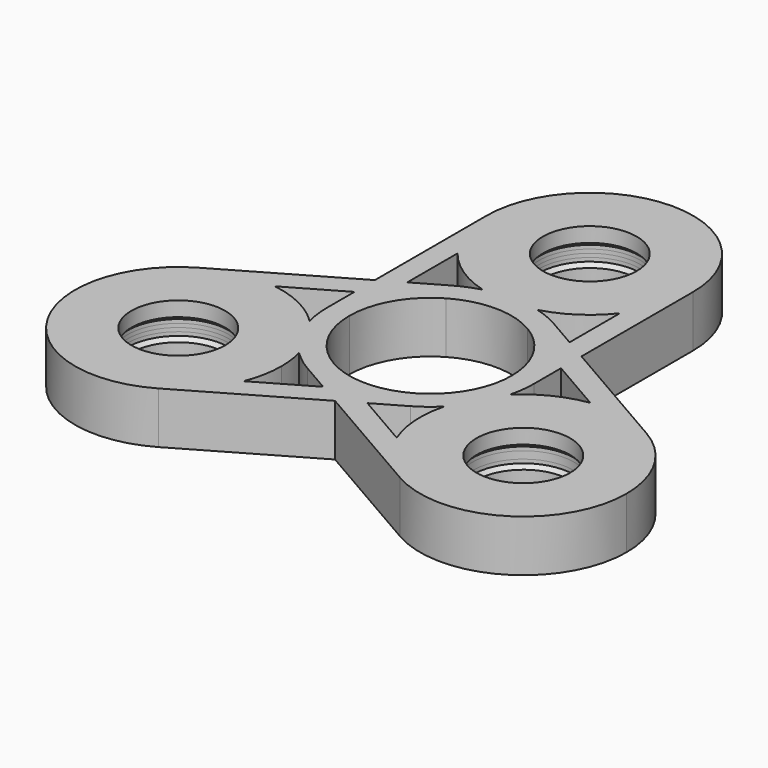
from build123d import *

# Parameters (mm, degrees)
F0_R         = 6.85
F0_R_2       = 6.35
F1_DEPTH     = 3.5
F2_DEPTH     = 0.5
F3_S5_R      = 6.85
F3_T6_DEPTH  = 12
F3_S11_R     = 6.85
F3_T12_DEPTH = 12
F3_S17_R     = 6.85
F3_T18_DEPTH = 12
F3_S23_R     = 6.85
F3_T24_DEPTH = 12
F3_S29_R     = 6.85
F3_T30_DEPTH = 12
F3_S35_R     = 6.85
F3_T36_DEPTH = 12


# Not quite as in the source:
# - a fillet or chamfer that OpenCascade refuses, or shapes differently, is made with other operations: its cross-section is extruded or revolved along the edge and cut away or added


with BuildPart() as f1:
    # F0 (on Top) → F1 (new body, symmetric)
    with BuildSketch(Plane.XY):
        with BuildLine():
            ThreePointArc((-11, 27), (0, 16), (11, 27))
            ThreePointArc((11, 27), (0, 38), (-11, 27))
        make_face()
        with Locations((0, 27)):
            Circle(F0_R, mode=Mode.SUBTRACT)
        with BuildLine():
            ThreePointArc((-28.882686, -3.973721), (-32.908965, -19), (-17.882686, -23.026279))
            ThreePointArc((-17.882686, -23.026279), (-13.856406, -19), (-12.382686, -13.5))
            ThreePointArc((-12.382686, -13.5), (-17.882686, -3.973721), (-28.882686, -3.973721))
        make_face()
        with Locations((-23.382686, -13.5)):
            Circle(F0_R, mode=Mode.SUBTRACT)
        with BuildLine():
            ThreePointArc((34.382686, -13.5), (32.908965, -8), (28.882686, -3.973721))
            ThreePointArc((28.882686, -3.973721), (13.856406, -8), (17.882686, -23.026279))
            ThreePointArc((17.882686, -23.026279), (28.882686, -23.026279), (34.382686, -13.5))
        make_face()
        with Locations((23.382686, -13.5)):
            Circle(F0_R, mode=Mode.SUBTRACT)
        with BuildLine():
            Line((11, 27), (11, 18.339746))
            ThreePointArc((11, 18.339746), (13.228757, 22.417424), (14, 27))
            ThreePointArc((14, 27), (0, 41), (-14, 27))
            ThreePointArc((-14, 27), (-13.228757, 22.417424), (-11, 18.339746))
            Line((-11, 18.339746), (-11, 27))
            ThreePointArc((-11, 27), (0, 38), (11, 27))
        make_face()
        with BuildLine():
            ThreePointArc((-16.382686, -25.624356), (-12.799681, -22.665151), (-10.382686, -18.696152))
            Line((-10.382686, -18.696152), (-17.882686, -23.026279))
            ThreePointArc((-17.882686, -23.026279), (-32.908965, -19), (-28.882686, -3.973721))
            Line((-28.882686, -3.973721), (-21.382686, 0.356406))
            ThreePointArc((-21.382686, 0.356406), (-26.028437, 0.247727), (-30.382686, -1.375644))
            ThreePointArc((-30.382686, -1.375644), (-35.507042, -20.5), (-16.382686, -25.624356))
        make_face()
        with BuildLine():
            ThreePointArc((30.382686, -1.375644), (26.028437, 0.247727), (21.382686, 0.356406))
            Line((21.382686, 0.356406), (28.882686, -3.973721))
            ThreePointArc((28.882686, -3.973721), (32.908965, -8), (34.382686, -13.5))
            ThreePointArc((34.382686, -13.5), (28.882686, -23.026279), (17.882686, -23.026279))
            Line((17.882686, -23.026279), (10.382686, -18.696152))
            ThreePointArc((10.382686, -18.696152), (12.799681, -22.665151), (16.382686, -25.624356))
            ThreePointArc((16.382686, -25.624356), (30.382686, -25.624356), (37.382686, -13.5))
            ThreePointArc((37.382686, -13.5), (35.507042, -6.5), (30.382686, -1.375644))
        make_face()
        with Locations((0, 27)):
            Circle(F0_R)
        with Locations((0, 27)):
            Circle(F0_R_2, mode=Mode.SUBTRACT)
        with Locations((-23.382686, -13.5)):
            Circle(F0_R)
        with Locations((-23.382686, -13.5)):
            Circle(F0_R_2, mode=Mode.SUBTRACT)
        with Locations((23.382686, -13.5)):
            Circle(F0_R)
        with Locations((23.382686, -13.5)):
            Circle(F0_R_2, mode=Mode.SUBTRACT)
        with BuildLine():
            ThreePointArc((-3.708099, 13.5), (0, 14), (3.708099, 13.5))
            ThreePointArc((3.708099, 13.5), (7.741953, 15.335431), (11, 18.339746))
            Line((11, 18.339746), (11, 27))
            ThreePointArc((11, 27), (0, 16), (-11, 27))
            Line((-11, 27), (-11, 18.339746))
            ThreePointArc((-11, 18.339746), (-7.741953, 15.335431), (-3.708099, 13.5))
        make_face()
        with BuildLine():
            ThreePointArc((-9.382686, -13.5), (-9.496803, -11.716113), (-9.837293, -9.961308))
            ThreePointArc((-9.837293, -9.961308), (-12.124356, -7), (-13.545393, -3.538692))
            ThreePointArc((-13.545393, -3.538692), (-17.151849, -0.962988), (-21.382686, 0.356406))
            Line((-21.382686, 0.356406), (-28.882686, -3.973721))
            ThreePointArc((-28.882686, -3.973721), (-17.882686, -3.973721), (-12.382686, -13.5))
            ThreePointArc((-12.382686, -13.5), (-13.856406, -19), (-17.882686, -23.026279))
            Line((-17.882686, -23.026279), (-10.382686, -18.696152))
            ThreePointArc((-10.382686, -18.696152), (-9.634959, -16.145751), (-9.382686, -13.5))
        make_face()
        with BuildLine():
            ThreePointArc((21.382686, 0.356406), (17.151849, -0.962988), (13.545393, -3.538692))
            ThreePointArc((13.545393, -3.538692), (12.124356, -7), (9.837293, -9.961308))
            ThreePointArc((9.837293, -9.961308), (9.409897, -14.372443), (10.382686, -18.696152))
            Line((10.382686, -18.696152), (17.882686, -23.026279))
            ThreePointArc((17.882686, -23.026279), (13.856406, -8), (28.882686, -3.973721))
            Line((28.882686, -3.973721), (21.382686, 0.356406))
        make_face()
        with BuildLine():
            ThreePointArc((-5.5, 9.526279), (0, 11), (5.5, 9.526279))
            Line((5.5, 9.526279), (11, 6.350853))
            Line((11, 6.350853), (11, 8.660254))
            ThreePointArc((11, 8.660254), (9.165151, 10.583005), (7, 12.124356))
            ThreePointArc((7, 12.124356), (5.39805, 12.917471), (3.708099, 13.5))
            ThreePointArc((3.708099, 13.5), (0, 13), (-3.708099, 13.5))
            ThreePointArc((-3.708099, 13.5), (-5.39805, 12.917471), (-7, 12.124356))
            ThreePointArc((-7, 12.124356), (-9.165151, 10.583005), (-11, 8.660254))
            Line((-11, 8.660254), (-11, 6.350853))
            Line((-11, 6.350853), (-5.5, 9.526279))
        make_face()
        with BuildLine():
            Line((11, 6.350853), (11, 0))
            ThreePointArc((11, 0), (9.526279, -5.5), (5.5, -9.526279))
            Line((5.5, -9.526279), (0, -12.701706))
            Line((0, -12.701706), (2, -13.856406))
            ThreePointArc((2, -13.856406), (4.582576, -13.228757), (7, -12.124356))
            ThreePointArc((7, -12.124356), (8.487833, -11.133584), (9.837293, -9.961308))
            ThreePointArc((9.837293, -9.961308), (11.25833, -6.5), (13.545393, -3.538692))
            ThreePointArc((13.545393, -3.538692), (13.885883, -1.783887), (14, 0))
            ThreePointArc((14, 0), (13.747727, 2.645751), (13, 5.196152))
            Line((13, 5.196152), (11, 6.350853))
        make_face()
        with BuildLine():
            Line((0, -12.701706), (-5.5, -9.526279))
            ThreePointArc((-5.5, -9.526279), (-9.526279, -5.5), (-11, 0))
            Line((-11, 0), (-11, 6.350853))
            Line((-11, 6.350853), (-13, 5.196152))
            ThreePointArc((-13, 5.196152), (-13.747727, 2.645751), (-14, 0))
            ThreePointArc((-14, 0), (-13.885883, -1.783887), (-13.545393, -3.538692))
            ThreePointArc((-13.545393, -3.538692), (-11.25833, -6.5), (-9.837293, -9.961308))
            ThreePointArc((-9.837293, -9.961308), (-8.487833, -11.133584), (-7, -12.124356))
            ThreePointArc((-7, -12.124356), (-4.582576, -13.228757), (-2, -13.856406))
            Line((-2, -13.856406), (0, -12.701706))
        make_face()
        with BuildLine():
            Line((-14, 8.082904), (-11, 9.814955))
            Line((-11, 9.814955), (-11, 18.339746))
            ThreePointArc((-11, 18.339746), (-13.228757, 22.417424), (-14, 27))
            Line((-14, 27), (-14, 8.082904))
        make_face()
        with BuildLine():
            Line((-21.382686, 0.356406), (-14, 4.618802))
            Line((-14, 4.618802), (-14, 8.082904))
            Line((-14, 8.082904), (-30.382686, -1.375644))
            ThreePointArc((-30.382686, -1.375644), (-26.028437, 0.247727), (-21.382686, 0.356406))
        make_face()
        with BuildLine():
            Line((0, -16.165808), (-3, -14.433757))
            Line((-3, -14.433757), (-10.382686, -18.696152))
            ThreePointArc((-10.382686, -18.696152), (-12.799681, -22.665151), (-16.382686, -25.624356))
            Line((-16.382686, -25.624356), (0, -16.165808))
        make_face()
        with BuildLine():
            Line((10.382686, -18.696152), (3, -14.433757))
            Line((3, -14.433757), (0, -16.165808))
            Line((0, -16.165808), (16.382686, -25.624356))
            ThreePointArc((16.382686, -25.624356), (12.799681, -22.665151), (10.382686, -18.696152))
        make_face()
        with BuildLine():
            Line((14, 8.082904), (14, 4.618802))
            Line((14, 4.618802), (21.382686, 0.356406))
            ThreePointArc((21.382686, 0.356406), (26.028437, 0.247727), (30.382686, -1.375644))
            Line((30.382686, -1.375644), (14, 8.082904))
        make_face()
        with BuildLine():
            Line((11, 18.339746), (11, 9.814955))
            Line((11, 9.814955), (14, 8.082904))
            Line((14, 8.082904), (14, 27))
            ThreePointArc((14, 27), (13.228757, 22.417424), (11, 18.339746))
        make_face()
        with BuildLine():
            Line((-14, 4.618802), (-13, 5.196152))
            ThreePointArc((-13, 5.196152), (-12.124356, 7), (-11, 8.660254))
            Line((-11, 8.660254), (-11, 9.814955))
            Line((-11, 9.814955), (-14, 8.082904))
            Line((-14, 8.082904), (-14, 4.618802))
        make_face()
        with BuildLine():
            Line((11, 9.814955), (11, 8.660254))
            ThreePointArc((11, 8.660254), (12.124356, 7), (13, 5.196152))
            Line((13, 5.196152), (14, 4.618802))
            Line((14, 4.618802), (14, 8.082904))
            Line((14, 8.082904), (11, 9.814955))
        make_face()
        with BuildLine():
            ThreePointArc((2, -13.856406), (0, -14), (-2, -13.856406))
            Line((-2, -13.856406), (-3, -14.433757))
            Line((-3, -14.433757), (0, -16.165808))
            Line((0, -16.165808), (3, -14.433757))
            Line((3, -14.433757), (2, -13.856406))
        make_face()
        with BuildLine():
            ThreePointArc((-11, 0), (-9.526279, 5.5), (-5.5, 9.526279))
            Line((-5.5, 9.526279), (-11, 6.350853))
            Line((-11, 6.350853), (-11, 0))
        make_face()
        with BuildLine():
            ThreePointArc((5.5, 9.526279), (9.526279, 5.5), (11, 0))
            Line((11, 0), (11, 6.350853))
            Line((11, 6.350853), (5.5, 9.526279))
        make_face()
        with BuildLine():
            Line((0, -12.701706), (5.5, -9.526279))
            ThreePointArc((5.5, -9.526279), (0, -11), (-5.5, -9.526279))
            Line((-5.5, -9.526279), (0, -12.701706))
        make_face()
        with BuildLine():
            ThreePointArc((-3.708099, 13.5), (0, 13), (3.708099, 13.5))
            ThreePointArc((3.708099, 13.5), (0, 14), (-3.708099, 13.5))
        make_face()
        with BuildLine():
            ThreePointArc((-13.545393, -3.538692), (-12.124356, -7), (-9.837293, -9.961308))
            ThreePointArc((-9.837293, -9.961308), (-11.25833, -6.5), (-13.545393, -3.538692))
        make_face()
        with BuildLine():
            ThreePointArc((9.837293, -9.961308), (12.124356, -7), (13.545393, -3.538692))
            ThreePointArc((13.545393, -3.538692), (11.25833, -6.5), (9.837293, -9.961308))
        make_face()
        with BuildLine():
            Line((-13, 5.196152), (-11, 6.350853))
            Line((-11, 6.350853), (-11, 8.660254))
            ThreePointArc((-11, 8.660254), (-12.124356, 7), (-13, 5.196152))
        make_face()
        with BuildLine():
            Line((11, 8.660254), (11, 6.350853))
            Line((11, 6.350853), (13, 5.196152))
            ThreePointArc((13, 5.196152), (12.124356, 7), (11, 8.660254))
        make_face()
        with BuildLine():
            Line((2, -13.856406), (0, -12.701706))
            Line((0, -12.701706), (-2, -13.856406))
            ThreePointArc((-2, -13.856406), (0, -14), (2, -13.856406))
        make_face()
        with BuildLine():
            Line((-11, 9.814955), (-11, 8.660254))
            ThreePointArc((-11, 8.660254), (-9.165151, 10.583005), (-7, 12.124356))
            Line((-7, 12.124356), (-11, 9.814955))
        make_face()
        with BuildLine():
            ThreePointArc((-14, 0), (-13.747727, 2.645751), (-13, 5.196152))
            Line((-13, 5.196152), (-14, 4.618802))
            Line((-14, 4.618802), (-14, 0))
        make_face()
        with BuildLine():
            ThreePointArc((7, 12.124356), (9.165151, 10.583005), (11, 8.660254))
            Line((11, 8.660254), (11, 9.814955))
            Line((11, 9.814955), (7, 12.124356))
        make_face()
        with BuildLine():
            ThreePointArc((7, -12.124356), (4.582576, -13.228757), (2, -13.856406))
            Line((2, -13.856406), (3, -14.433757))
            Line((3, -14.433757), (7, -12.124356))
        make_face()
        with BuildLine():
            Line((14, 4.618802), (13, 5.196152))
            ThreePointArc((13, 5.196152), (13.747727, 2.645751), (14, 0))
            Line((14, 0), (14, 4.618802))
        make_face()
        with BuildLine():
            Line((-3, -14.433757), (-2, -13.856406))
            ThreePointArc((-2, -13.856406), (-4.582576, -13.228757), (-7, -12.124356))
            Line((-7, -12.124356), (-3, -14.433757))
        make_face()
    extrude(amount=F1_DEPTH, both=True)

    # F0 (on Top) → F2 (cut, symmetric)
    with BuildSketch(Plane.XY):
        with Locations((0, 27)):
            Circle(F0_R)
        with Locations((0, 27)):
            Circle(F0_R_2, mode=Mode.SUBTRACT)
        with Locations((-23.382686, -13.5)):
            Circle(F0_R)
        with Locations((-23.382686, -13.5)):
            Circle(F0_R_2, mode=Mode.SUBTRACT)
        with Locations((23.382686, -13.5)):
            Circle(F0_R)
        with Locations((23.382686, -13.5)):
            Circle(F0_R_2, mode=Mode.SUBTRACT)
    extrude(amount=F2_DEPTH, both=True, mode=Mode.SUBTRACT)

    # F3: chamfer of 1 on 6 edges, made by hand


with BuildPart() as f3_tool2:
    # F3_s3 → F3_t4 (revolve)
    with BuildSketch(Plane.XZ.offset(-27)):
        Polygon((6.35, 1.5), (7.35, 0.5), (6.35, 0.5), align=None)
    revolve(axis=Axis((0, 27, 0.5), (0, 0, 1)))

    # F3_s5 → F3_t6 (intersect, symmetric)
    with BuildSketch(Plane.XY.offset(1)):
        with Locations((0, 27)):
            Circle(F3_S5_R)
    extrude(amount=F3_T6_DEPTH, both=True, mode=Mode.INTERSECT)


with BuildPart() as f1_1:
    add(f1.part)

    # F3_t1: cut F3_tool2
    add(f3_tool2.part, mode=Mode.SUBTRACT)


with BuildPart() as f3_tool8:
    # F3_s9 → F3_t10 (revolve)
    with BuildSketch(Plane.XZ.offset(-27)):
        Polygon((7.35, -0.5), (6.35, -1.5), (6.35, -0.5), align=None)
    revolve(axis=Axis((0, 27, -0.5), (0, 0, 1)))

    # F3_s11 → F3_t12 (intersect, symmetric)
    with BuildSketch(Plane.XY.offset(-1)):
        with Locations((0, 27)):
            Circle(F3_S11_R)
    extrude(amount=F3_T12_DEPTH, both=True, mode=Mode.INTERSECT)


with BuildPart() as f1_2:
    add(f1_1.part)

    # F3_t7: cut F3_tool8
    add(f3_tool8.part, mode=Mode.SUBTRACT)


with BuildPart() as f3_tool14:
    # F3_s15 → F3_t16 (revolve)
    with BuildSketch(Plane.XZ.offset(13.5)):
        Polygon((29.732686, 1.5), (30.732686, 0.5), (29.732686, 0.5), align=None)
    revolve(axis=Axis((23.382686, -13.5, 0.5), (0, 0, 1)))

    # F3_s17 → F3_t18 (intersect, symmetric)
    with BuildSketch(Plane.XY.offset(1)):
        with Locations((23.382686, -13.5)):
            Circle(F3_S17_R)
    extrude(amount=F3_T18_DEPTH, both=True, mode=Mode.INTERSECT)


with BuildPart() as f1_3:
    add(f1_2.part)

    # F3_t13: cut F3_tool14
    add(f3_tool14.part, mode=Mode.SUBTRACT)


with BuildPart() as f3_tool20:
    # F3_s21 → F3_t22 (revolve)
    with BuildSketch(Plane.XZ.offset(13.5)):
        Polygon((30.732686, -0.5), (29.732686, -1.5), (29.732686, -0.5), align=None)
    revolve(axis=Axis((23.382686, -13.5, -0.5), (0, 0, 1)))

    # F3_s23 → F3_t24 (intersect, symmetric)
    with BuildSketch(Plane.XY.offset(-1)):
        with Locations((23.382686, -13.5)):
            Circle(F3_S23_R)
    extrude(amount=F3_T24_DEPTH, both=True, mode=Mode.INTERSECT)


with BuildPart() as f1_4:
    add(f1_3.part)

    # F3_t19: cut F3_tool20
    add(f3_tool20.part, mode=Mode.SUBTRACT)


with BuildPart() as f3_tool26:
    # F3_s27 → F3_t28 (revolve)
    with BuildSketch(Plane.XZ.offset(13.5)):
        Polygon((-16.032686, -0.5), (-17.032686, -1.5), (-17.032686, -0.5), align=None)
    revolve(axis=Axis((-23.382686, -13.5, -0.5), (0, 0, 1)))

    # F3_s29 → F3_t30 (intersect, symmetric)
    with BuildSketch(Plane.XY.offset(-1)):
        with Locations((-23.382686, -13.5)):
            Circle(F3_S29_R)
    extrude(amount=F3_T30_DEPTH, both=True, mode=Mode.INTERSECT)


with BuildPart() as f1_5:
    add(f1_4.part)

    # F3_t25: cut F3_tool26
    add(f3_tool26.part, mode=Mode.SUBTRACT)


with BuildPart() as f3_tool32:
    # F3_s33 → F3_t34 (revolve)
    with BuildSketch(Plane.XZ.offset(13.5)):
        Polygon((-17.032686, 1.5), (-16.032686, 0.5), (-17.032686, 0.5), align=None)
    revolve(axis=Axis((-23.382686, -13.5, 0.5), (0, 0, 1)))

    # F3_s35 → F3_t36 (intersect, symmetric)
    with BuildSketch(Plane.XY.offset(1)):
        with Locations((-23.382686, -13.5)):
            Circle(F3_S35_R)
    extrude(amount=F3_T36_DEPTH, both=True, mode=Mode.INTERSECT)


with BuildPart() as f1_6:
    add(f1_5.part)

    # F3_t31: cut F3_tool32
    add(f3_tool32.part, mode=Mode.SUBTRACT)


solid = f1_6.part
